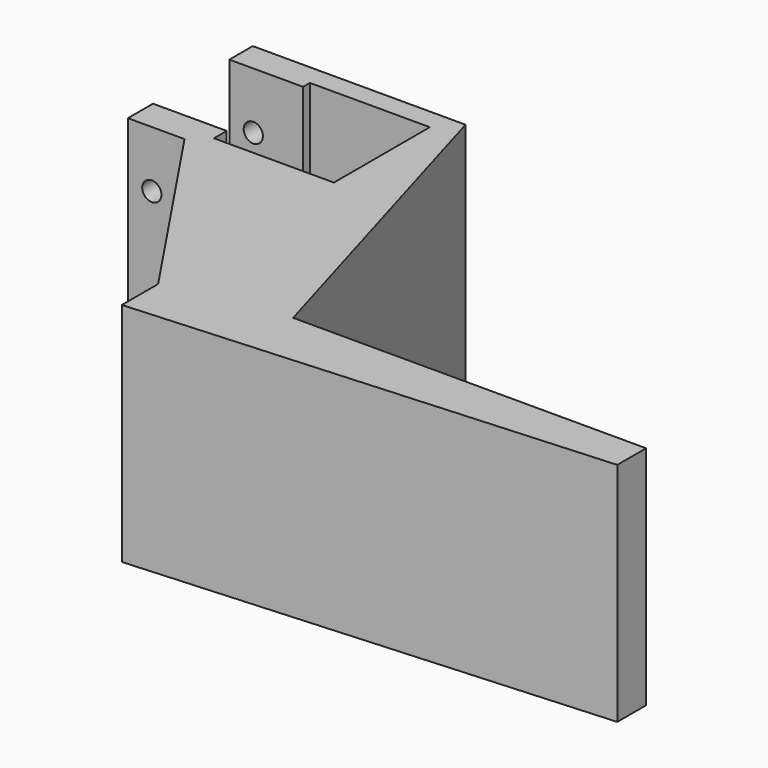
from build123d import *

# Parameters (mm, degrees)
F1_DEPTH = 50
F3_D     = 4.25


# Not quite as in the source:
# - a feature names something its author has since deleted; it is built from what else it names


with BuildPart() as f1:
    # F0 (on Top) → F1 (new body)
    with BuildSketch(Plane.XY):
        Polygon((-30.2708722231, 4.5814236456), (-30.2708722231, 0), (-30.2708722231, -1.8863187066), (-26.5, -1.8863187066), (-26.5, 0), (0, 0), (0, -26.5), (-26.5, -26.5), (-26.5, -22.9706130922), (-30.2708722231, -22.9706130922), (-30.2708722231, -26.5), (-30.2708722231, -29.9115763544), (0, -29.9115763544), (4.2217531975, -29.9115763544), (4.2217531975, 0), (4.2217531975, 4.5814236456), align=None)
        Polygon((-30.2708722231, -1.8863187066), (-30.2708722231, 0), (-30.2708722231, 4.5814236456), (-42.7924469113, 4.5814236456), (-42.7924469113, -1.8863187066), align=None)
        Polygon((-42.7924469113, -29.9115763544), (-30.2708722231, -29.9115763544), (-30.2708722231, -26.5), (-30.2708722231, -22.9706130922), (-42.7924469113, -22.9706130922), align=None)
        Polygon((0, -75.0411301851), (0, -29.9115763544), (-30.2708722231, -29.9115763544), align=None)
        Polygon((104.0906682611, -70.3669339418), (26.0842684656, -70.3669339418), (4.2217531975, -70.3669339418), (4.2217531975, -29.9115763544), (0, -29.9115763544), (0, -75.0411301851), (0, -85.0630626082), (104.0906682611, -78.3288473744), (104.0906682611, -75.0411301851), align=None)
        Polygon((26.0842684656, -70.3669339418), (4.2217531975, 4.5814236456), (4.2217531975, 0), (4.2217531975, -29.9115763544), (4.2217531975, -70.3669339418), align=None)
    extrude(amount=F1_DEPTH)

    # F3 (through all)
    with Locations(Plane(origin=(0, 4.5814236456, 0), x_dir=(-1, 0, 0), z_dir=(0, 1, 0))):
        with Locations((37.5032611191, 37.5), (37.5032611191, 12.5)):
            Hole(F3_D / 2)


solid = f1.part
